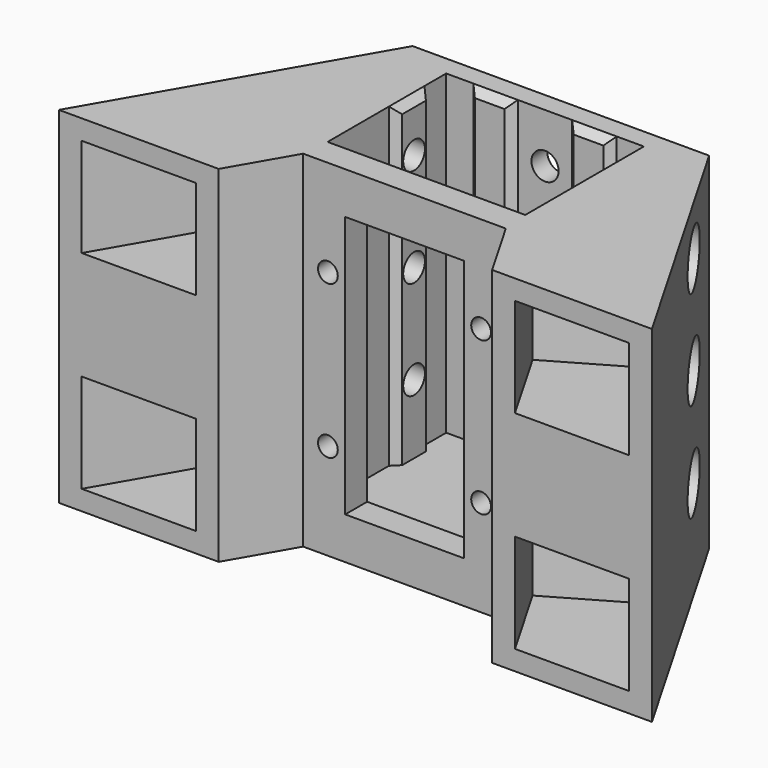
from build123d import *

# Parameters (mm, degrees)
F1_DEPTH       = 70
F2_W           = 40
F2_H           = 20
F3_DEPTH       = 64
F6_DEPTH       = 20
F9_DEPTH       = 20
F11_DEPTH      = 70.001
F12_W          = 24
F12_H          = 53
F13_DEPTH      = 15.5455173281
F14_R          = 2
F15_DEPTH      = 15.5455173281
F16_DEPTH      = 10
F17_W          = 1.5
F17_H          = 9
F17_W_2        = 9
F17_H_2        = 1.5
F18_DEPTH      = 64
F19_SIZE       = 1.49999
F20_R          = 2.75
F21_DEPTH      = 41.501
F21_DEPTH_BACK = 78.501
F24_R          = 5.5
F25_DEPTH      = 36.001
F26_R          = 5.5
F27_DEPTH      = 36.001
F28_R          = 2.75
F29_DEPTH      = 4.001


# Not quite as in the source:
# - a fillet or chamfer is up to 0.001 mm smaller than in the source, because OpenCascade refuses the exact size


with BuildPart() as f1:
    # F0 (on Top) → F1 (new body)
    with BuildSketch(Plane.XY):
        Polygon((30, 51.9615242271), (0, 0), (120, 0), (90, 51.9615242271), align=None)
    extrude(amount=F1_DEPTH)

    # F2 (on face) → F3 (cut)
    with BuildSketch(Plane.XY.offset(70)):
        with Locations((60, 37.9615242271)):
            Rectangle(F2_W, F2_H)
    extrude(amount=-F3_DEPTH, mode=Mode.SUBTRACT)

    # F5 (on offset) → F6 (cut)
    with BuildSketch(Plane.XY.offset(4)):
        Polygon((19.6188021535, 25.9807621135), (4.6188021535, 0), (27.7128129211, 0), (36.9393102292, 15.9807621135), align=None)
        Polygon((100.3811978465, 25.9807621135), (83.0606897708, 15.9807621135), (92.2871870789, 0), (115.3811978465, 0), align=None)
    extrude(amount=F6_DEPTH, mode=Mode.SUBTRACT)

    # F8 (on offset) → F9 (cut)
    with BuildSketch(Plane.XY.offset(66)):
        Polygon((19.6188021535, 25.9807621135), (4.6188021535, 0), (27.7128129211, 0), (36.9393102292, 15.9807621135), align=None)
        Polygon((100.3811978465, 25.9807621135), (83.0606897708, 15.9807621135), (92.2871870789, 0), (115.3811978465, 0), align=None)
    extrude(amount=-F9_DEPTH, mode=Mode.SUBTRACT)

    # F10 (on face) → F11 (cut, through all)
    with BuildSketch(Plane.XY.offset(70)):
        Polygon((39.5, 12.416006899), (32.3316150746, 0), (87.6683849254, 0), (80.5, 12.416006899), align=None)
    extrude(amount=-F11_DEPTH, mode=Mode.SUBTRACT)

    # F12 (on face) → F13 (cut, through all)
    with BuildSketch(Plane.XZ.offset(-12.416006899)):
        with Locations((60, 35)):
            Rectangle(F12_W, F12_H)
    extrude(amount=-F13_DEPTH, mode=Mode.SUBTRACT)

    # F14 (on face) → F15 (cut, through all)
    with BuildSketch(Plane.XZ.offset(-12.416006899)):
        with Locations((44.5, 50.5)):
            Circle(F14_R)
        with Locations((44.5, 19.5)):
            Circle(F14_R)
        with Locations((75.5, 19.5)):
            Circle(F14_R)
        with Locations((75.5, 50.5)):
            Circle(F14_R)
    extrude(amount=-F15_DEPTH, mode=Mode.SUBTRACT)

    # F16 (cut): a face of the model
    f16_faces = [f1.faces().sort_by_distance(p)[0] for p in [
        (40.7547184906, 27.9615242271, 38),
    ]]
    extrude(f16_faces, amount=-F16_DEPTH, mode=Mode.SUBTRACT)

    # F17 (on face) → F18 (join, through all)
    with BuildSketch(Plane.XY.offset(70)):
        with Locations((40.75, 37.9615242271)):
            Rectangle(F17_W, F17_H)
        with Locations((50, 47.2115242271)):
            Rectangle(F17_W_2, F17_H_2)
        with Locations((79.25, 37.9615242271)):
            Rectangle(F17_W, F17_H)
        with Locations((70, 47.2115242271)):
            Rectangle(F17_W_2, F17_H_2)
    extrude(amount=-F18_DEPTH)

    # F19 (size 1.5 in the source; OpenCascade refuses exactly that, so slightly less here)
    f19_edges = [f1.edges().sort_by_distance(p)[0] for p in [
        (54.5, 46.461524, 38),
        (45.5, 46.461524, 38),
        (50, 46.461524, 70),
        (41.5, 37.961524, 70),
        (41.5, 33.461524, 38),
        (65.5, 46.461524, 38),
        (74.5, 46.461524, 38),
        (78.5, 33.461524, 38),
        (78.5, 42.461524, 38),
        (70, 46.461524, 70),
        (78.5, 37.961524, 70),
        (41.5, 42.461524, 38),
    ]]
    chamfer(f19_edges, length=F19_SIZE)

    # F20 (on face) → F21 (cut, two sides)
    with BuildSketch(Plane(origin=(78.5, 0, 0), x_dir=(0, -1, 0), z_dir=(-1, 0, 0))) as f21_sk:
        with Locations((-37.9615242271, 60)):
            Circle(F20_R)
        with Locations((-37.9615242271, 40)):
            Circle(F20_R)
        with Locations((-37.9615242271, 20)):
            Circle(F20_R)
    extrude(amount=-F21_DEPTH, mode=Mode.SUBTRACT)
    extrude(f21_sk.sketch, amount=F21_DEPTH_BACK, mode=Mode.SUBTRACT)

    # F24 (on offset) → F25 (cut, through all)
    with BuildSketch(Plane(origin=(84, 0, 0), x_dir=(0, -1, 0), z_dir=(-1, 0, 0))):
        with Locations((-37.9615242271, 60)):
            Circle(F24_R)
        with Locations((-37.9615242271, 40)):
            Circle(F24_R)
        with Locations((-37.9615242271, 20)):
            Circle(F24_R)
    extrude(amount=-F25_DEPTH, mode=Mode.SUBTRACT)

    # F26 (on offset) → F27 (cut, through all)
    with BuildSketch(Plane.YZ.offset(36)):
        with Locations((37.9615242271, 60)):
            Circle(F26_R)
        with Locations((37.9615242271, 40)):
            Circle(F26_R)
        with Locations((37.9615242271, 20)):
            Circle(F26_R)
    extrude(amount=-F27_DEPTH, mode=Mode.SUBTRACT)

    # F28 (on face) → F29 (cut, through all)
    with BuildSketch(Plane.XZ.offset(-47.9615242271)):
        with Locations((60, 60)):
            Circle(F28_R)
        with Locations((60, 40)):
            Circle(F28_R)
        with Locations((60, 20)):
            Circle(F28_R)
    extrude(amount=-F29_DEPTH, mode=Mode.SUBTRACT)


solid = f1.part
